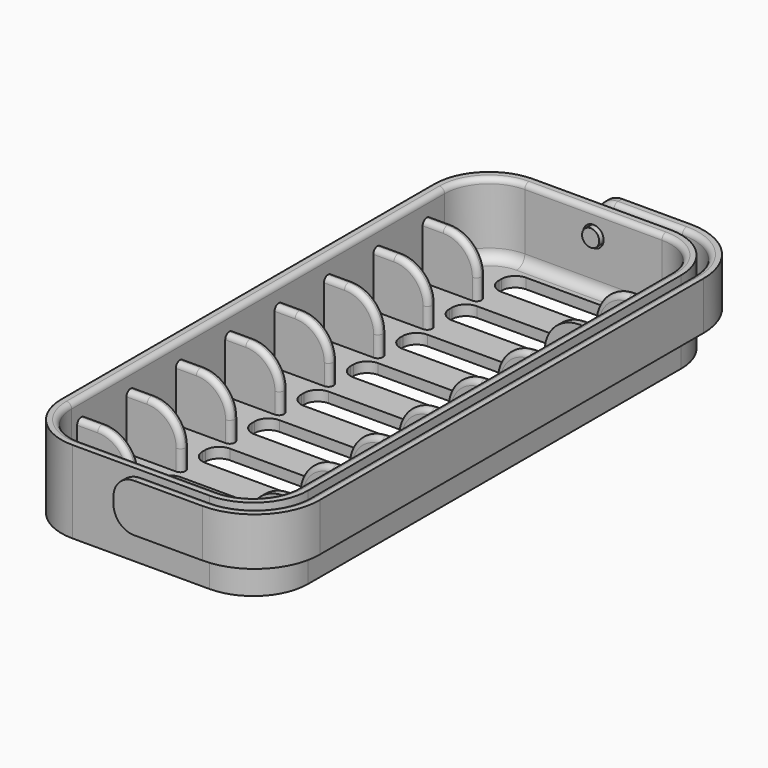
from build123d import *

# Parameters (mm, degrees)
F0_W      = 36
F0_H      = 84
F1_DEPTH  = 12
F2_R      = 8
F3_T      = -1.5
F4_W      = 8
F4_H      = 1.5
F5_DEPTH  = 8
F6_R      = 5
F7_W      = 20
F7_H      = 4.5
F8_DEPTH  = 25
F9_R      = 2
F10_R     = 1.5
F12_R     = 0.74999
F16_DEPTH = 7
F18_R     = 3
F19_R     = 0.75
F17_R     = 1.5
F20_DEPTH = 100
F21_R     = 1.5166818765
F22_DEPTH = 1.5
F23_R     = 1.25
F24_DEPTH = 3
F25_R     = 1.5097591608
F26_DEPTH = 1.5
F27_R     = 1.25
F28_DEPTH = 3


# Not quite as in the source:
# - two fillets or chamfers of one size are made in one step
# - a fillet or chamfer is up to 0.001 mm smaller than in the source, because OpenCascade refuses the exact size


with BuildPart() as f1:
    # F0 (on Top) → F1 (new body)
    with BuildSketch(Plane.XY):
        Rectangle(F0_W, F0_H)
    extrude(amount=F1_DEPTH)

    # F2
    f2_edges = [f1.edges().sort_by_distance(p)[0] for p in [
        (18, 42, 6),
        (18, -42, 6),
        (-18, -42, 6),
        (-18, 42, 6),
    ]]
    fillet(f2_edges, radius=F2_R)

    # F3
    f3_openings = [f1.faces().sort_by_distance(p)[0] for p in [
        (0, 0, 12),
    ]]
    offset(amount=F3_T, openings=f3_openings)

    # F4 (on face) → F5 (join)
    with BuildSketch(Plane.XY.offset(1.5)):
        with Locations((-12.5, 30.75)):
            Rectangle(F4_W, F4_H)
        with Locations((-12.5, 21.75)):
            Rectangle(F4_W, F4_H)
        with Locations((-12.5, 12.75)):
            Rectangle(F4_W, F4_H)
        with Locations((-12.5, 3.75)):
            Rectangle(F4_W, F4_H)
        with Locations((-12.5, -5.25)):
            Rectangle(F4_W, F4_H)
        with Locations((-12.5, -14.25)):
            Rectangle(F4_W, F4_H)
        with Locations((-12.5, -23.25)):
            Rectangle(F4_W, F4_H)
        with Locations((-12.5, -32.25)):
            Rectangle(F4_W, F4_H)
        with Locations((12.5, 30.75)):
            Rectangle(F4_W, F4_H)
        with Locations((12.5, 21.75)):
            Rectangle(F4_W, F4_H)
        with Locations((12.5, 12.75)):
            Rectangle(F4_W, F4_H)
        with Locations((12.5, 3.75)):
            Rectangle(F4_W, F4_H)
        with Locations((12.5, -5.25)):
            Rectangle(F4_W, F4_H)
        with Locations((12.5, -14.25)):
            Rectangle(F4_W, F4_H)
        with Locations((12.5, -23.25)):
            Rectangle(F4_W, F4_H)
        with Locations((12.5, -32.25)):
            Rectangle(F4_W, F4_H)
    extrude(amount=F5_DEPTH)

    # F6
    f6_edges = [f1.edges().sort_by_distance(p)[0] for p in [
        (-8.5, -32.25, 9.5),
        (-8.5, -23.25, 9.5),
        (-8.5, -14.25, 9.5),
        (-8.5, -5.25, 9.5),
        (-8.5, 3.75, 9.5),
        (-8.5, 12.75, 9.5),
        (-8.5, 21.75, 9.5),
        (-8.5, 30.75, 9.5),
        (8.5, 30.75, 9.5),
        (8.5, 21.75, 9.5),
        (8.5, 12.75, 9.5),
        (8.5, 3.75, 9.5),
        (8.5, -5.25, 9.5),
        (8.5, -14.25, 9.5),
        (8.5, -23.25, 9.5),
        (8.5, -32.25, 9.5),
    ]]
    fillet(f6_edges, radius=F6_R)

    # F7 (on face) → F8 (cut)
    with BuildSketch(Plane.XY.offset(1.5)):
        with Locations((0, 36)):
            Rectangle(F7_W, F7_H)
        with Locations((0, 27)):
            Rectangle(F7_W, F7_H)
        with Locations((0, 18)):
            Rectangle(F7_W, F7_H)
        with Locations((0, 9)):
            Rectangle(F7_W, F7_H)
        Rectangle(F7_W, F7_H)
        with Locations((0, -9)):
            Rectangle(F7_W, F7_H)
        with Locations((0, -18)):
            Rectangle(F7_W, F7_H)
        with Locations((0, -27)):
            Rectangle(F7_W, F7_H)
        with Locations((0, -36)):
            Rectangle(F7_W, F7_H)
    extrude(amount=-F8_DEPTH, mode=Mode.SUBTRACT)

    # F9
    f9_edges = [f1.edges().sort_by_distance(p)[0] for p in [
        (-10, 38.25, 0.75),
        (10, 38.25, 0.75),
        (10, 29.25, 0.75),
        (10, 20.25, 0.75),
        (10, 11.25, 0.75),
        (10, 2.25, 0.75),
        (10, -6.75, 0.75),
        (10, -15.75, 0.75),
        (10, -24.75, 0.75),
        (10, -38.25, 0.75),
        (10, -29.25, 0.75),
        (10, -20.25, 0.75),
        (10, -11.25, 0.75),
        (10, -2.25, 0.75),
        (10, 6.75, 0.75),
        (10, 15.75, 0.75),
        (10, 33.75, 0.75),
        (10, 24.75, 0.75),
        (-10, 20.25, 0.75),
        (-10, 29.25, 0.75),
        (-10, 11.25, 0.75),
        (-10, 2.25, 0.75),
        (-10, -6.75, 0.75),
        (-10, -15.75, 0.75),
        (-10, -20.25, 0.75),
        (-10, -29.25, 0.75),
        (-10, -38.25, 0.75),
        (-10, -11.25, 0.75),
        (-10, -2.25, 0.75),
        (-10, -33.75, 0.75),
        (-10, -24.75, 0.75),
        (-10, 6.75, 0.75),
        (-10, 15.75, 0.75),
        (-10, 24.75, 0.75),
        (-10, 33.75, 0.75),
        (10, -33.75, 0.75),
    ]]
    fillet(f9_edges, radius=F9_R)

    # F10
    f10_edges = [f1.edges().sort_by_distance(p)[0] for p in [
        (16.5, 26.25, 1.5),
        (16.5, 17.25, 1.5),
        (16.5, 8.25, 1.5),
        (16.5, -0.75, 1.5),
        (16.5, -9.75, 1.5),
        (16.5, -18.75, 1.5),
        (16.5, -27.75, 1.5),
        (14.596194, 38.596194, 1.5),
        (16.5, 32.75, 1.5),
        (0, 40.5, 1.5),
        (-14.596194, 38.596194, 1.5),
        (-16.5, 32.75, 1.5),
        (-16.5, 26.25, 1.5),
        (-16.5, 17.25, 1.5),
        (-16.5, 8.25, 1.5),
        (-16.5, -0.75, 1.5),
        (-16.5, -9.75, 1.5),
        (-16.5, -18.75, 1.5),
        (-16.5, -27.75, 1.5),
        (16.5, -33.5, 1.5),
        (14.596194, -38.596194, 1.5),
        (0, -40.5, 1.5),
        (-16.5, -33.5, 1.5),
        (-14.596194, -38.596194, 1.5),
    ]]
    fillet(f10_edges, radius=F10_R)

    # F12 (radius 0.75 in the source; OpenCascade refuses exactly that, so slightly less here)
    f12_edges = [f1.edges().sort_by_distance(p)[0] for p in [
        (-9.964466, 3, 8.035534),
        (-9.964466, 12, 8.035534),
        (-9.964466, 13.5, 8.035534),
        (-9.964466, 21, 8.035534),
        (-9.964466, 22.5, 8.035534),
        (-9.964466, 4.5, 8.035534),
        (-9.964466, 30, 8.035534),
        (-9.964466, 31.5, 8.035534),
        (9.964466, 31.5, 8.035534),
        (9.964466, 30, 8.035534),
        (9.964466, 22.5, 8.035534),
        (9.964466, 13.5, 8.035534),
        (9.964466, 12, 8.035534),
        (9.964466, 4.5, 8.035534),
        (9.964466, 3, 8.035534),
        (9.964466, -4.5, 8.035534),
        (9.964466, -6, 8.035534),
        (9.964466, -13.5, 8.035534),
        (9.964466, -15, 8.035534),
        (9.964466, -22.5, 8.035534),
        (9.964466, -24, 8.035534),
        (9.964466, -31.5, 8.035534),
        (-9.964466, -33, 8.035534),
        (-9.964466, -24, 8.035534),
        (-9.964466, -22.5, 8.035534),
        (-9.964466, -31.5, 8.035534),
        (-9.964466, -15, 8.035534),
        (-9.964466, -6, 8.035534),
        (-9.964466, -13.5, 8.035534),
        (-9.964466, -4.5, 8.035534),
        (-16.5, 0, 12),
    ]]
    fillet(f12_edges, radius=F12_R)

    # F17 (on face) → F20 (cut)
    with BuildSketch(Plane(origin=(0, 44.5, 0), x_dir=(-1, 0, 0), z_dir=(0, 1, 0))):
        with Locations((0, 8.5)):
            Circle(F17_R)
    extrude(amount=-F20_DEPTH, mode=Mode.SUBTRACT)


with BuildPart() as f16:
    # F15 (on offset) → F16 (new body)
    with BuildSketch(Plane.XY.offset(5)):
        with BuildLine():
            Line((-2, 43), (0, 43))
            Line((0, 43), (11, 43))
            ThreePointArc((11, 43), (16.6568542495, 40.6568542495), (19, 35))
            Line((19, 35), (19, -35))
            ThreePointArc((19, -35), (16.6568542495, -40.6568542495), (11, -43))
            Line((11, -43), (0, -43))
            Line((0, -43), (-2, -43))
            Line((-2, -43), (-2, -44.5))
            Line((-2, -44.5), (0, -44.5))
            Line((0, -44.5), (11, -44.5))
            ThreePointArc((11, -44.5), (17.7175144213, -41.7175144213), (20.5, -35))
            Line((20.5, -35), (20.5, 35))
            ThreePointArc((20.5, 35), (17.7175144213, 41.7175144213), (11, 44.5))
            Line((11, 44.5), (0, 44.5))
            Line((0, 44.5), (-2, 44.5))
            Line((-2, 44.5), (-2, 43))
        make_face()
    extrude(amount=F16_DEPTH)

    # F18
    f18_edges = [f16.edges().sort_by_distance(p)[0] for p in [
        (-2, -43.75, 12),
        (-2, -43.75, 5),
        (-2, 43.75, 12),
        (-2, 43.75, 5),
    ]]
    fillet(f18_edges, radius=F18_R)

    # F19
    f19_edges = [f16.edges().sort_by_distance(p)[0] for p in [
        (19, 0, 12),
        (6, 43, 12),
        (16.656854, 40.656854, 12),
        (16.656854, -40.656854, 12),
        (6, -43, 12),
        (-1.12132, 43, 11.12132),
        (-1.12132, 43, 5.87868),
        (6, 43, 5),
        (16.656854, 40.656854, 5),
        (19, 0, 5),
        (16.656854, -40.656854, 5),
        (-1.12132, -43, 11.12132),
        (6, -43, 5),
        (-1.12132, -43, 5.87868),
    ]]
    fillet(f19_edges, radius=F19_R)

    # F21 (on face) → F22 (join)
    with BuildSketch(Plane.XZ.offset(44.5)):
        with Locations((0, 8.5)):
            Circle(F21_R)
    extrude(amount=-F22_DEPTH)

    # F23 (on face) → F24 (join)
    with BuildSketch(Plane(origin=(0, -43, 0), x_dir=(-1, 0, 0), z_dir=(0, 1, 0))):
        with Locations((0, 8.5)):
            Circle(F23_R)
    extrude(amount=F24_DEPTH)

    # F25 (on face) → F26 (join)
    with BuildSketch(Plane(origin=(0, 44.5, 0), x_dir=(-1, 0, 0), z_dir=(0, 1, 0))):
        with Locations((0, 8.5)):
            Circle(F25_R)
    extrude(amount=-F26_DEPTH)

    # F27 (on face) → F28 (join)
    with BuildSketch(Plane.XZ.offset(-43)):
        with Locations((0, 8.5)):
            Circle(F27_R)
    extrude(amount=F28_DEPTH)


solid = Compound([f1.part, f16.part])
